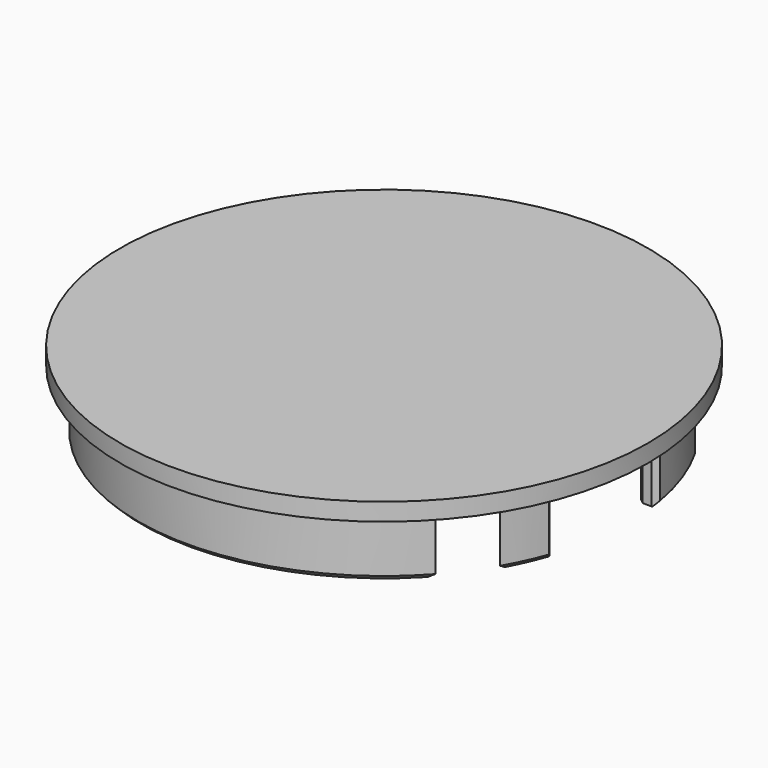
from build123d import *

# Parameters (mm, degrees)
F0_R         = 30
F1_DEPTH     = 2
F2_R         = 27.95
F3_DEPTH     = 7
F4_T         = -2
F5_W         = 13
F5_H         = 10
F6_DEPTH     = 30
F7_T1_DEPTH  = 7.3004746493
F7_T3_DEPTH  = 6.5918643954
F7_T5_DEPTH  = 6.4134609486
F7_T7_DEPTH  = 7.0163816712
F7_T12_ANGLE = 11.2783830284
F7_T17_ANGLE = 20.9875744089
F7_T22_ANGLE = 22.6619870068
F7_T27_ANGLE = 12.1533364168
F7_T30_ANGLE = 338.3067764097
F7_T35_ANGLE = 11.2783830284
F7_T39_DEPTH = 7.0163816712
F7_T47_DEPTH = 7.3004746493
F7_T52_ANGLE = 20.9875744089
F7_T59_ANGLE = 22.6619870068
F7_T63_DEPTH = 6.4134609486
F7_T70_ANGLE = 12.1533364168
F7_T74_DEPTH = 6.5918643954
F8_R         = 4.5
F9_DEPTH     = 25


# Not quite as in the source:
# - a fillet or chamfer that OpenCascade refuses, or shapes differently, is made with other operations: its cross-section is extruded or revolved along the edge and cut away or added


with BuildPart() as f1:
    # F0 (on Top) → F1 (new body)
    with BuildSketch(Plane.XY):
        Circle(F0_R)
    extrude(amount=F1_DEPTH)

    # F2 (on face) → F3 (join)
    with BuildSketch(Plane(origin=(0, 0, 0), x_dir=(1, 0, 0), z_dir=(0, 0, -1))):
        Circle(F2_R)
    extrude(amount=F3_DEPTH)

    # F4
    f4_openings = [f1.faces().sort_by_distance(p)[0] for p in [
        (0, 0, -7),
    ]]
    offset(amount=F4_T, openings=f4_openings, kind=Kind.INTERSECTION)

    # F5 (on Right) → F6 (cut)
    with BuildSketch(Plane.YZ):
        with Locations((-2.3, -6.5)):
            Rectangle(F5_W, F5_H)
    extrude(amount=F6_DEPTH, mode=Mode.SUBTRACT)

    # F7: chamfer of 0.5 on 9 edges, made by hand

    # F7_s2 → F7_t1 (cut)
    with BuildSketch(Plane.XY.offset(-8.8004746493)):
        with BuildLine():
            Line((26.2970147419, -9.4693989071), (25.8265851401, -8.8))
            Line((25.8265851401, -8.8), (26.5285223863, -8.8))
            ThreePointArc((26.5285223863, -8.8), (26.4129758895, -9.1409630052), (26.2970147419, -9.4693989071))
        make_face()
    extrude(amount=F7_T1_DEPTH, mode=Mode.SUBTRACT)

    # F7_s4 → F7_t3 (cut)
    with BuildSketch(Plane.XY.offset(-8.0918643954)):
        with BuildLine():
            Line((26.0290702869, 4.2), (25.5370273703, 4.6111531191))
            ThreePointArc((25.5370273703, 4.6111531191), (25.5719745626, 4.4132320321), (25.6078601215, 4.2))
            Line((25.6078601215, 4.2), (26.0290702869, 4.2))
        make_face()
    extrude(amount=F7_T3_DEPTH, mode=Mode.SUBTRACT)

    # F7_s6 → F7_t5 (cut)
    with BuildSketch(Plane.XY.offset(-7.9134609486)):
        with BuildLine():
            Line((24.7611086182, -8.8), (24.2930347312, -9.1241965974))
            ThreePointArc((24.2930347312, -9.1241965974), (24.3504005172, -8.9699774052), (24.4123431895, -8.8))
            Line((24.4123431895, -8.8), (24.7611086182, -8.8))
        make_face()
    extrude(amount=F7_T5_DEPTH, mode=Mode.SUBTRACT)

    # F7_s8 → F7_t7 (cut)
    with BuildSketch(Plane.XY.offset(-8.5163816712)):
        with BuildLine():
            Line((27.5372554008, 4.7856102004), (27.0446390251, 4.2))
            Line((27.0446390251, 4.2), (27.6326346916, 4.2))
            ThreePointArc((27.6326346916, 4.2), (27.585450674, 4.4994900946), (27.5372554008, 4.7856102004))
        make_face()
    extrude(amount=F7_T7_DEPTH, mode=Mode.SUBTRACT)


with BuildPart() as f7_tool10:
    # F7_s11 → F7_t12 (revolve)
    with BuildSketch(Plane.XZ):
        Polygon((27.95, -1), (27.45, -1.5), (27.95, -1.5), align=None)
    revolve(axis=Axis((0, 0, -1.5), (0, 0, 1)), revolution_arc=F7_T12_ANGLE)

    split(bisect_by=Plane.XZ.offset(-4.2), keep=Keep.TOP)


with BuildPart() as f1_1:
    add(f1.part)

    # F7_t9: cut F7_tool10
    add(f7_tool10.part, mode=Mode.SUBTRACT)


with BuildPart() as f7_tool15:
    # F7_s16 → F7_t17 (revolve)
    with BuildSketch(Plane(origin=(0, 0, 0), x_dir=(0, 0, 1), z_dir=(-0.3581654779, -0.9336581229, 0))):
        Polygon((-1, -27.95), (-1.5, -27.45), (-1.5, -27.95), align=None)
    revolve(axis=Axis((0, 0, -1.5), (0, 0, 1)), revolution_arc=F7_T17_ANGLE)

    split(bisect_by=Plane.XZ.offset(8.8), keep=Keep.BOTTOM)


with BuildPart() as f1_2:
    add(f1_1.part)

    # F7_t14: cut F7_tool15
    add(f7_tool15.part, mode=Mode.SUBTRACT)


with BuildPart() as f7_tool20:
    # F7_s21 → F7_t22 (revolve)
    with BuildSketch(Plane(origin=(0, 0, 0), x_dir=(0, 0, 1), z_dir=(-0.3852938978, -0.9227939165, 0))):
        Polygon((-1.5, -26.45), (-1, -25.95), (-1.5, -25.95), align=None)
    revolve(axis=Axis((0, 0, -1.5), (0, 0, 1)), revolution_arc=F7_T22_ANGLE)

    split(bisect_by=Plane.XZ.offset(8.8), keep=Keep.BOTTOM)


with BuildPart() as f1_3:
    add(f1_2.part)

    # F7_t19: cut F7_tool20
    add(f7_tool20.part, mode=Mode.SUBTRACT)


with BuildPart() as f7_tool25:
    # F7_s26 → F7_t27 (revolve)
    with BuildSketch(Plane.XZ):
        Polygon((26.45, -1.5), (25.95, -1), (25.95, -1.5), align=None)
    revolve(axis=Axis((0, 0, -1.5), (0, 0, 1)), revolution_arc=F7_T27_ANGLE)

    split(bisect_by=Plane.XZ.offset(-4.2), keep=Keep.TOP)


with BuildPart() as f1_4:
    add(f1_3.part)

    # F7_t24: cut F7_tool25
    add(f7_tool25.part, mode=Mode.SUBTRACT)

    # F7_s29 → F7_t30 (revolve, cut)
    with BuildSketch(Plane(origin=(0, 0, 0), x_dir=(0, 0, 1), z_dir=(0.2706204465, 0.9626861243, 0))):
        Polygon((-6.5, 27.95), (-7, 27.45), (-7, 27.95), align=None)
    revolve(axis=Axis((0, 0, -7), (0, 0, -1)), revolution_arc=F7_T30_ANGLE, mode=Mode.SUBTRACT)


with BuildPart() as f7_tool33:
    # F7_s34 → F7_t35 (revolve)
    with BuildSketch(Plane.XZ):
        Polygon((27.95, -1), (27.45, -1.5), (27.95, -1.5), align=None)
    revolve(axis=Axis((0, 0, -1.5), (0, 0, 1)), revolution_arc=F7_T35_ANGLE)

    split(bisect_by=Plane.XZ.offset(-4.2), keep=Keep.BOTTOM)


with BuildPart() as f7_tool37:
    # F7_s38 → F7_t39 (new body)
    with BuildSketch(Plane.XY.offset(-7)):
        with BuildLine():
            Line((27.5372554008, 4.7856102004), (27.0446390251, 4.2))
            Line((27.0446390251, 4.2), (27.6326346916, 4.2))
            ThreePointArc((27.6326346916, 4.2), (27.585450674, 4.4994900946), (27.5372554008, 4.7856102004))
        make_face()
    extrude(amount=F7_T39_DEPTH)

    split(bisect_by=Plane.XY, keep=Keep.BOTTOM)

    split(bisect_by=Plane.XY.offset(-1.5), keep=Keep.TOP)


with BuildPart() as f7_tool33_1:
    add(f7_tool33.part)

    # F7_t42: intersect F7_tool37
    add(f7_tool37.part, mode=Mode.INTERSECT)


with BuildPart() as f1_5:
    add(f1_4.part)

    # F7_t31: cut F7_tool33
    add(f7_tool33_1.part, mode=Mode.SUBTRACT)


with BuildPart() as f7_tool45:
    # F7_s46 → F7_t47 (new body)
    with BuildSketch(Plane.XY.offset(-7)):
        with BuildLine():
            Line((26.2970147419, -9.4693989071), (25.8265851401, -8.8))
            Line((25.8265851401, -8.8), (26.5285223863, -8.8))
            ThreePointArc((26.5285223863, -8.8), (26.4129758895, -9.1409630052), (26.2970147419, -9.4693989071))
        make_face()
    extrude(amount=F7_T47_DEPTH)

    split(bisect_by=Plane.XY, keep=Keep.BOTTOM)

    split(bisect_by=Plane.XY.offset(-1.5), keep=Keep.TOP)


with BuildPart() as f7_tool50:
    # F7_s51 → F7_t52 (revolve)
    with BuildSketch(Plane(origin=(0, 0, 0), x_dir=(0, 0, 1), z_dir=(-0.3581654779, -0.9336581229, 0))):
        Polygon((-1, -27.95), (-1.5, -27.45), (-1.5, -27.95), align=None)
    revolve(axis=Axis((0, 0, -1.5), (0, 0, 1)), revolution_arc=F7_T52_ANGLE)

    split(bisect_by=Plane.XZ.offset(8.8), keep=Keep.TOP)


with BuildPart() as f7_tool45_1:
    add(f7_tool45.part)

    # F7_t54: intersect F7_tool50
    add(f7_tool50.part, mode=Mode.INTERSECT)


with BuildPart() as f1_6:
    add(f1_5.part)

    # F7_t43: cut F7_tool45
    add(f7_tool45_1.part, mode=Mode.SUBTRACT)


with BuildPart() as f7_tool57:
    # F7_s58 → F7_t59 (revolve)
    with BuildSketch(Plane(origin=(0, 0, 0), x_dir=(0, 0, 1), z_dir=(-0.3852938978, -0.9227939165, 0))):
        Polygon((-1.5, -26.45), (-1, -25.95), (-1.5, -25.95), align=None)
    revolve(axis=Axis((0, 0, -1.5), (0, 0, 1)), revolution_arc=F7_T59_ANGLE)

    split(bisect_by=Plane.XZ.offset(8.8), keep=Keep.TOP)


with BuildPart() as f7_tool61:
    # F7_s62 → F7_t63 (new body)
    with BuildSketch(Plane.XY.offset(-7)):
        with BuildLine():
            Line((24.7611086182, -8.8), (24.2930347312, -9.1241965974))
            ThreePointArc((24.2930347312, -9.1241965974), (24.3504005172, -8.9699774052), (24.4123431895, -8.8))
            Line((24.4123431895, -8.8), (24.7611086182, -8.8))
        make_face()
    extrude(amount=F7_T63_DEPTH)

    split(bisect_by=Plane.XY.offset(-1.5), keep=Keep.TOP)


with BuildPart() as f7_tool57_1:
    add(f7_tool57.part)

    # F7_t65: intersect F7_tool61
    add(f7_tool61.part, mode=Mode.INTERSECT)


with BuildPart() as f1_7:
    add(f1_6.part)

    # F7_t55: cut F7_tool57
    add(f7_tool57_1.part, mode=Mode.SUBTRACT)


with BuildPart() as f7_tool68:
    # F7_s69 → F7_t70 (revolve)
    with BuildSketch(Plane.XZ):
        Polygon((26.45, -1.5), (25.95, -1), (25.95, -1.5), align=None)
    revolve(axis=Axis((0, 0, -1.5), (0, 0, 1)), revolution_arc=F7_T70_ANGLE)

    split(bisect_by=Plane.XZ.offset(-4.2), keep=Keep.BOTTOM)


with BuildPart() as f7_tool72:
    # F7_s73 → F7_t74 (new body)
    with BuildSketch(Plane.XY.offset(-7)):
        with BuildLine():
            Line((26.0290702869, 4.2), (25.5370273703, 4.6111531191))
            ThreePointArc((25.5370273703, 4.6111531191), (25.5719745626, 4.4132320321), (25.6078601215, 4.2))
            Line((25.6078601215, 4.2), (26.0290702869, 4.2))
        make_face()
    extrude(amount=F7_T74_DEPTH)

    split(bisect_by=Plane.XY.offset(-1.5), keep=Keep.TOP)


with BuildPart() as f7_tool68_1:
    add(f7_tool68.part)

    # F7_t76: intersect F7_tool72
    add(f7_tool72.part, mode=Mode.INTERSECT)


with BuildPart() as f1_8:
    add(f1_7.part)

    # F7_t66: cut F7_tool68
    add(f7_tool68_1.part, mode=Mode.SUBTRACT)

    # F8 (on face) → F9 (cut)
    with BuildSketch(Plane.XY):
        with Locations((19.798791036, -14.3004134297)):
            Circle(F8_R)
        with Locations((-19.798791036, -14.3004134297)):
            Circle(F8_R)
        with Locations((19.798791036, 14.3004134297)):
            Circle(F8_R)
        with Locations((-19.798791036, 14.3004134297)):
            Circle(F8_R)
    extrude(amount=-F9_DEPTH, mode=Mode.SUBTRACT)


solid = f1_8.part
